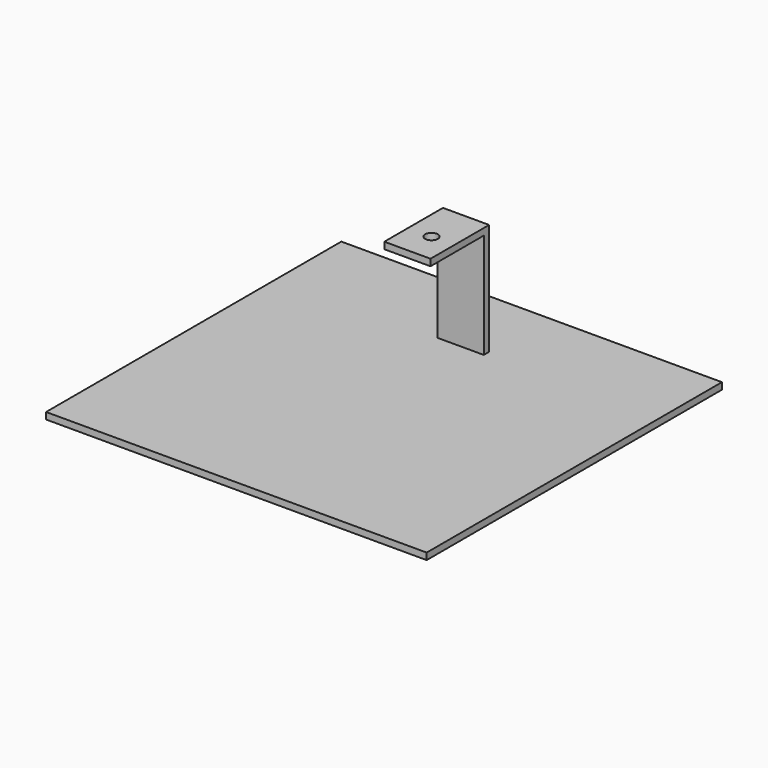
from build123d import *

# Parameters (mm, degrees)
F0_W          = 114.3
F0_H          = 110.8363599028
F2_DEPTH      = 2
F1_E1_W       = 13.8702858239
F1_E1_H       = 35.56
F3_DEPTH      = 2
F5_E4_W       = 13.8702858239
F5_E4_H       = 20
F6_DEPTH      = 2
F7_R          = 1.905
F8_DEPTH      = 6.858
F8_DEPTH_BACK = 2.032


with BuildPart() as f2:
    # F0 (on Top) → F2 (new body)
    with BuildSketch(Plane.XY):
        Rectangle(F0_W, F0_H)
    extrude(amount=F2_DEPTH)

    # F1_E1 (on explicit) → F3 (join)
    with BuildSketch(Plane(origin=(-8.9655527845, 33.3296358585, 0), x_dir=(1, 0, 0), z_dir=(0, -1, 0))):
        with Locations((6.935142912, 17.78)):
            Rectangle(F1_E1_W, F1_E1_H)
    extrude(amount=F3_DEPTH)

    # F5_E4 (on explicit) → F6 (join)
    with BuildSketch(Plane(origin=(-8.9655527845, 31.3296358585, 35.56), x_dir=(1, 0, 0), z_dir=(0, 0, -1))):
        with Locations((6.935142912, 10)):
            Rectangle(F5_E4_W, F5_E4_H)
    extrude(amount=F6_DEPTH)

    # F7 (on face) → F8 (cut, two sides)
    with BuildSketch(Plane(origin=(0, 0, 35.56), x_dir=(1, 0, 0), z_dir=(0, 0, -1))) as f8_sk:
        with Locations((-1.9456632435, -20.2625636011)):
            Circle(F7_R)
    extrude(amount=F8_DEPTH, mode=Mode.SUBTRACT)
    extrude(f8_sk.sketch, amount=-F8_DEPTH_BACK, mode=Mode.SUBTRACT)


solid = f2.part
